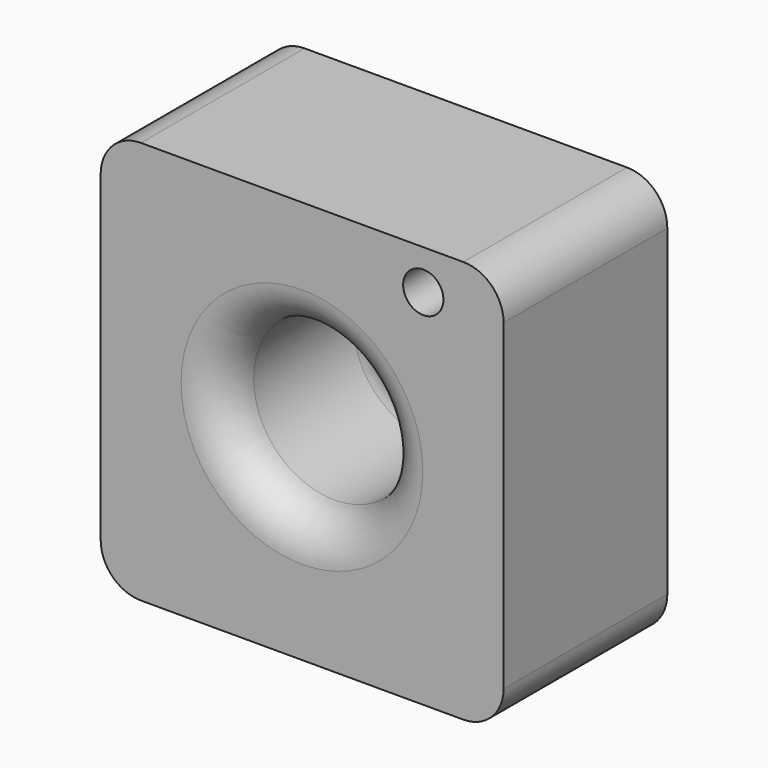
from build123d import *

# Parameters (mm, degrees)
F0_W     = 50
F0_H     = 50
F1_DEPTH = 25.4
F3_D     = 20
F4_R     = 5
F6_D     = 5


with BuildPart() as f1:
    # F0 (on Front) → F1 (new body)
    with BuildSketch(Plane.XZ):
        with Locations((25, 25)):
            Rectangle(F0_W, F0_H)
    extrude(amount=F1_DEPTH)

    # F3 (through all)
    with Locations(Plane.XZ.offset(25.4)):
        with Locations((24.9791759998, 25.4528727382)):
            Hole(F3_D / 2)

    # F4
    f4_edges = [f1.edges().sort_by_distance(p)[0] for p in [
        (50, -12.7, 50),
        (50, -12.7, 0),
        (0, -12.7, 50),
        (0, -12.7, 0),
        (14.979176, 0, 25.452873),
        (14.979176, -25.4, 25.452873),
    ]]
    fillet(f4_edges, radius=F4_R)

    # F6 (through all)
    with Locations(Plane.XZ.offset(25.4)):
        with Locations((40.0353602501, 45.0723162054)):
            Hole(F6_D / 2)


solid = f1.part
